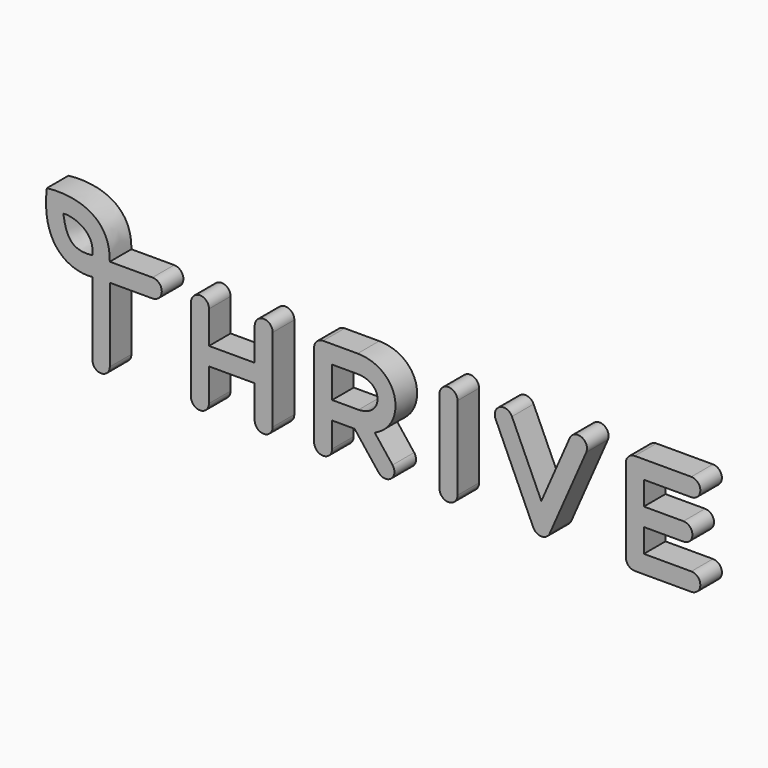
from build123d import *

# Parameters (mm, degrees)
F1_DEPTH = 3
F0_W     = 5.0755630732
F0_H     = 2


# Not quite as in the source:
# - ends of sketch curves that miss each other by under 0.0002 mm in the source are joined


with BuildPart() as f1:
    # F0 (on Front) → F1 (new body)
    with BuildSketch(Plane.XZ):
        with BuildLine():
            ThreePointArc((5.9279855341, 1.2211229187), (6.8863565102, 0.2627519425), (7.8447274864, 1.2211229187))
            Line((7.8447274864, 1.2211229187), (7.8447274864, 9.4423424453))
            Line((7.8447274864, 9.4423424453), (12.5910351053, 9.4423424453))
            ThreePointArc((12.5910351053, 9.4423424453), (13.6175910011, 10.4688983411), (12.5910351053, 11.4954542369))
            Line((12.5910351053, 11.4954542369), (7.8447274864, 11.4954542369))
            add(Edge.make_bspline(
                [(7.8447274864, 11.4954542369), (7.917419076, 15.7590787858), (4.1587534361, 16.7871546), (0.8551732753, 16.4163727313)],
                knots=[0, 0, 0, 0, 8.5480586625, 8.5480586625, 8.5480586625, 8.5480586625], degree=3))
            add(Edge.make_bspline(
                [(5.9279855341, 9.382002987), (3.6362486426, 9.1018620878), (0.1472634031, 10.568135418), (0.8551732753, 16.4163727313)],
                knots=[0, 0, 0, 0, 8.6727032644, 8.6727032644, 8.6727032644, 8.6727032644], degree=3))
            Line((5.9279855341, 9.382002987), (5.9279855341, 1.2211229187))
        make_face()
        with BuildLine():
            add(Edge.make_bspline(
                [(5.8948188089, 11.4954542369), (6.2487735413, 13.8040473685), (3.7710885517, 14.6467331797), (2.6755135041, 14.5287569612)],
                knots=[0, 0, 0, 0, 4.4232173882, 4.4232173882, 4.4232173882, 4.4232173882], degree=3))
            add(Edge.make_bspline(
                [(5.8948188089, 11.4954542369), (3.3160033636, 11.1748687923), (2.9789034743, 12.8096789122), (2.6755135041, 14.5287569612)],
                knots=[0, 0, 0, 0, 4.4232173882, 4.4232173882, 4.4232173882, 4.4232173882], degree=3))
        make_face(mode=Mode.SUBTRACT)
    extrude(amount=F1_DEPTH)


with BuildPart() as f1b:
    # F0 (on Front) → F1, piece 2 (new body)
    with BuildSketch(Plane.XZ):
        with BuildLine():
            ThreePointArc((17.8618747741, 6.8450106299), (17.1547679929, 6.552117411), (16.8618747741, 5.8450106299))
            ThreePointArc((16.8618747741, 5.8450106299), (17.1547679929, 5.1379038487), (17.8618747741, 4.8450106299))
            Line((17.8618747741, 4.8450106299), (18.8618747741, 4.8450106299))
            Line((18.8618747741, 4.8450106299), (18.8618747741, 6.8450106299))
            Line((18.8618747741, 6.8450106299), (17.8618747741, 6.8450106299))
        make_face()
        with BuildLine():
            Line((24.9374378473, 4.8450106299), (23.9374378473, 4.8450106299))
            Line((23.9374378473, 4.8450106299), (23.9374378473, 1.2211229187))
            ThreePointArc((23.9374378473, 1.2211229187), (24.9374378473, 0.2211229187), (25.9374378473, 1.2211229187))
            Line((25.9374378473, 1.2211229187), (25.9374378473, 5.8450106299))
            ThreePointArc((25.9374378473, 5.8450106299), (25.6445446284, 5.1379038487), (24.9374378473, 4.8450106299))
        make_face()
        with Locations((21.3996563107, 5.8450106299)):
            Rectangle(F0_W, F0_H)
        with BuildLine():
            ThreePointArc((18.8618747741, 10.4688983411), (17.8618747741, 11.4688983411), (16.8618747741, 10.4688983411))
            Line((16.8618747741, 10.4688983411), (16.8618747741, 5.8450106299))
            ThreePointArc((16.8618747741, 5.8450106299), (17.1547679929, 6.552117411), (17.8618747741, 6.8450106299))
            Line((17.8618747741, 6.8450106299), (18.8618747741, 6.8450106299))
            Line((18.8618747741, 6.8450106299), (18.8618747741, 10.4688983411))
        make_face()
        with BuildLine():
            ThreePointArc((17.8618747741, 4.8450106299), (17.1547679929, 5.1379038487), (16.8618747741, 5.8450106299))
            Line((16.8618747741, 5.8450106299), (16.8618747741, 1.2211229187))
            ThreePointArc((16.8618747741, 1.2211229187), (17.8618747741, 0.2211229187), (18.8618747741, 1.2211229187))
            Line((18.8618747741, 1.2211229187), (18.8618747741, 4.8450106299))
            Line((18.8618747741, 4.8450106299), (17.8618747741, 4.8450106299))
        make_face()
        with BuildLine():
            Line((23.9374378473, 10.4688983411), (23.9374378473, 6.8450106299))
            Line((23.9374378473, 6.8450106299), (24.9374378473, 6.8450106299))
            ThreePointArc((24.9374378473, 6.8450106299), (25.6445446284, 6.552117411), (25.9374378473, 5.8450106299))
            Line((25.9374378473, 5.8450106299), (25.9374378473, 10.4688983411))
            ThreePointArc((25.9374378473, 10.4688983411), (24.9374378473, 11.4688983411), (23.9374378473, 10.4688983411))
        make_face()
        with BuildLine():
            Line((24.9374378473, 6.8450106299), (23.9374378473, 6.8450106299))
            Line((23.9374378473, 6.8450106299), (23.9374378473, 4.8450106299))
            Line((23.9374378473, 4.8450106299), (24.9374378473, 4.8450106299))
            ThreePointArc((24.9374378473, 4.8450106299), (25.6445446284, 5.1379038487), (25.9374378473, 5.8450106299))
            ThreePointArc((25.9374378473, 5.8450106299), (25.6445446284, 6.552117411), (24.9374378473, 6.8450106299))
        make_face()
    extrude(amount=F1_DEPTH)


with BuildPart() as f1c:
    # F0 (on Front) → F1, piece 3 (new body)
    with BuildSketch(Plane.XZ):
        with BuildLine():
            ThreePointArc((44.4577468336, 1.2211229187), (45.4577468336, 0.2211229187), (46.4577468336, 1.2211229187))
            Line((46.4577468336, 1.2211229187), (46.4577468336, 10.4688983411))
            ThreePointArc((46.4577468336, 10.4688983411), (45.4577468336, 11.4688983411), (44.4577468336, 10.4688983411))
            Line((44.4577468336, 10.4688983411), (44.4577468336, 1.2211229187))
        make_face()
    extrude(amount=F1_DEPTH)


with BuildPart() as f1d:
    # F0 (on Front) → F1, piece 4 (new body)
    with BuildSketch(Plane.XZ):
        with BuildLine():
            ThreePointArc((52.5072458972, 10.8813804322), (51.1837980962, 11.3798640509), (50.6853144775, 10.0564162499))
            Line((50.6853144775, 10.0564162499), (54.8726748835, 0.8086408275))
            ThreePointArc((54.8726748835, 0.8086408275), (54.7836581967, 1.2151894114), (54.8678441825, 1.6227657126))
            Line((54.8678441825, 1.6227657126), (55.7690644442, 3.6776619873))
            Line((55.7690644442, 3.6776619873), (52.5072458972, 10.8813804322))
        make_face()
        with BuildLine():
            Line((58.9236608627, 10.870541135), (55.7690644442, 3.6776619873))
            Line((55.7690644442, 3.6776619873), (56.6946063031, 1.6336050098))
            ThreePointArc((56.6946063031, 1.6336050098), (56.7836229899, 1.2270564259), (56.6994370041, 0.8194801247))
            Line((56.6994370041, 0.8194801247), (60.7552536843, 10.0672555471))
            ThreePointArc((60.7552536843, 10.0672555471), (60.2411000674, 11.3846947519), (58.9236608627, 10.870541135))
        make_face()
        with BuildLine():
            ThreePointArc((54.8678441825, 1.6227657126), (54.7836581967, 1.2151894114), (54.8726748835, 0.8086408275))
            ThreePointArc((54.8726748835, 0.8086408275), (55.7895741006, 0.2211405221), (56.6994370041, 0.8194801247))
            ThreePointArc((56.6994370041, 0.8194801247), (56.7836229899, 1.2270564259), (56.6946063031, 1.6336050098))
            Line((56.6946063031, 1.6336050098), (55.7690644442, 3.6776619873))
            Line((55.7690644442, 3.6776619873), (54.8678441825, 1.6227657126))
        make_face()
    extrude(amount=F1_DEPTH)


with BuildPart() as f1e:
    # F0 (on Front) → F1, piece 5 (new body)
    with BuildSketch(Plane.XZ):
        with BuildLine():
            Line((67.1533847451, 9.4688983411), (66.1533847451, 9.4688983411))
            ThreePointArc((66.1533847451, 9.4688983411), (65.4462779639, 9.7617915599), (65.1533847451, 10.4688983411))
            Line((65.1533847451, 10.4688983411), (65.1533847451, 5.8450106299))
            ThreePointArc((65.1533847451, 5.8450106299), (65.4462779639, 6.552117411), (66.1533847451, 6.8450106299))
            Line((66.1533847451, 6.8450106299), (67.1533847451, 6.8450106299))
            Line((67.1533847451, 6.8450106299), (67.1533847451, 9.4688983411))
        make_face()
        with BuildLine():
            Line((67.1533847451, 10.4688983411), (67.1533847451, 9.4688983411))
            Line((67.1533847451, 9.4688983411), (72.4234580994, 9.4688983411))
            ThreePointArc((72.4234580994, 9.4688983411), (73.4234580994, 10.4688983411), (72.4234580994, 11.4688983411))
            Line((72.4234580994, 11.4688983411), (66.1533847451, 11.4688983411))
            ThreePointArc((66.1533847451, 11.4688983411), (66.8604915263, 11.1760051222), (67.1533847451, 10.4688983411))
        make_face()
        with BuildLine():
            Line((71.5465247631, 6.8450106299), (67.1533847451, 6.8450106299))
            Line((67.1533847451, 6.8450106299), (67.1533847451, 4.8450106299))
            Line((67.1533847451, 4.8450106299), (71.5465247631, 4.8450106299))
            ThreePointArc((71.5465247631, 4.8450106299), (72.5465247631, 5.8450106299), (71.5465247631, 6.8450106299))
        make_face()
        with BuildLine():
            ThreePointArc((67.1533847451, 1.2211229187), (66.8604915263, 0.5140161375), (66.1533847451, 0.2211229187))
            Line((66.1533847451, 0.2211229187), (72.4234580994, 0.2211229187))
            ThreePointArc((72.4234580994, 0.2211229187), (73.4234580994, 1.2211229187), (72.4234580994, 2.2211229187))
            Line((72.4234580994, 2.2211229187), (67.1533847451, 2.2211229187))
            Line((67.1533847451, 2.2211229187), (67.1533847451, 1.2211229187))
        make_face()
        with BuildLine():
            ThreePointArc((66.1533847451, 6.8450106299), (65.4462779639, 6.552117411), (65.1533847451, 5.8450106299))
            ThreePointArc((65.1533847451, 5.8450106299), (65.4462779639, 5.1379038487), (66.1533847451, 4.8450106299))
            Line((66.1533847451, 4.8450106299), (67.1533847451, 4.8450106299))
            Line((67.1533847451, 4.8450106299), (67.1533847451, 6.8450106299))
            Line((67.1533847451, 6.8450106299), (66.1533847451, 6.8450106299))
        make_face()
        with BuildLine():
            ThreePointArc((66.1533847451, 4.8450106299), (65.4462779639, 5.1379038487), (65.1533847451, 5.8450106299))
            Line((65.1533847451, 5.8450106299), (65.1533847451, 1.2211229187))
            ThreePointArc((65.1533847451, 1.2211229187), (65.4462779639, 1.9282296998), (66.1533847451, 2.2211229187))
            Line((66.1533847451, 2.2211229187), (67.1533847451, 2.2211229187))
            Line((67.1533847451, 2.2211229187), (67.1533847451, 4.8450106299))
            Line((67.1533847451, 4.8450106299), (66.1533847451, 4.8450106299))
        make_face()
        with BuildLine():
            ThreePointArc((66.1533847451, 2.2211229187), (65.4462779639, 1.9282296998), (65.1533847451, 1.2211229187))
            ThreePointArc((65.1533847451, 1.2211229187), (65.4462779639, 0.5140161375), (66.1533847451, 0.2211229187))
            ThreePointArc((66.1533847451, 0.2211229187), (66.8604915263, 0.5140161375), (67.1533847451, 1.2211229187))
            Line((67.1533847451, 1.2211229187), (67.1533847451, 2.2211229187))
            Line((67.1533847451, 2.2211229187), (66.1533847451, 2.2211229187))
        make_face()
        with BuildLine():
            ThreePointArc((65.1533847451, 10.4688983411), (65.4462779639, 9.7617915599), (66.1533847451, 9.4688983411))
            Line((66.1533847451, 9.4688983411), (67.1533847451, 9.4688983411))
            Line((67.1533847451, 9.4688983411), (67.1533847451, 10.4688983411))
            ThreePointArc((67.1533847451, 10.4688983411), (66.8604915263, 11.1760051222), (66.1533847451, 11.4688983411))
            ThreePointArc((66.1533847451, 11.4688983411), (65.4462779639, 11.1760051222), (65.1533847451, 10.4688983411))
        make_face()
    extrude(amount=F1_DEPTH)


with BuildPart() as f1f:
    # F0 (on Front) → F1, piece 6 (new body)
    with BuildSketch(Plane.XZ):
        with BuildLine():
            ThreePointArc((30.5364226699, 1.2211229187), (31.5364226699, 0.2211229187), (32.5364226699, 1.2211229187))
            Line((32.5364226699, 1.2211229187), (32.5364226699, 4.0022602994))
            Line((32.5364226699, 4.0022602994), (35.0292300262, 4.0022602994))
            Line((35.0292300262, 4.0022602994), (37.6841082637, 0.610509659))
            ThreePointArc((37.6841082637, 0.610509659), (39.0748130113, 0.4410314307), (39.2442912396, 1.8317361783))
            Line((39.2442912396, 1.8317361783), (37.2624160319, 4.3636890228))
            add(Edge.make_bspline(
                [(35.3682806871, 11.4688983411), (36.0047684908, 11.457952021), (37.1712736186, 11.2425154442), (38.5277131215, 10.3972749102), (39.3744537744, 9.1750766328), (39.6676411305, 7.780445673), (39.4145740003, 6.3824201645), (38.6184785966, 5.1516953575), (37.754583761, 4.5694914405), (37.2624160319, 4.3636890228)],
                knots=[0, 0, 0, 0, 0.125, 0.25, 0.375, 0.5, 0.625, 0.75, 0.8727798803, 0.8727798803, 0.8727798803, 0.8727798803], degree=3))
            Line((35.3682806871, 11.4688983411), (31.5364226699, 11.4688983411))
            ThreePointArc((31.5364226699, 11.4688983411), (30.8293158887, 11.1760051222), (30.5364226699, 10.4688983411))
            Line((30.5364226699, 10.4688983411), (30.5364226699, 1.2211229187))
        make_face()
        with BuildLine():
            Line((32.5364226699, 6.0015435255), (32.5364226699, 9.4688983411))
            Line((32.5364226699, 9.4688983411), (35.3420294949, 9.4688983411))
            add(Edge.make_bspline(
                [(35.3420294949, 9.4688983411), (35.770598662, 9.4607038174), (36.4714047742, 9.3165116696), (37.1211796946, 8.8947736693), (37.4876230201, 8.3610140526), (37.6168150326, 7.7518956041), (37.5050546188, 7.1386772873), (37.1574531687, 6.5982897882), (36.5409989908, 6.170884027), (35.8768194338, 6.01679006), (35.467341449, 6.0015435255)],
                knots=[0.0007857187, 0.0007857187, 0.0007857187, 0.0007857187, 0.125, 0.25, 0.375, 0.5, 0.625, 0.75, 0.875, 1, 1, 1, 1], degree=3))
            Line((35.467341449, 6.0015435255), (32.5364226699, 6.0015435255))
        make_face(mode=Mode.SUBTRACT)
    extrude(amount=F1_DEPTH)


solid = Compound([f1.part, f1b.part, f1c.part, f1d.part, f1e.part, f1f.part])
